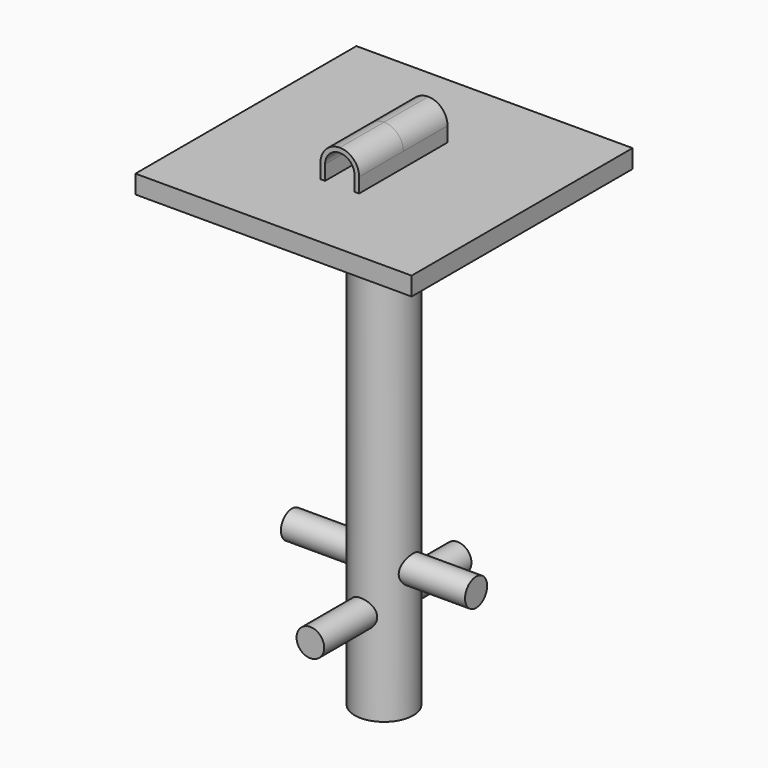
from build123d import *

# Parameters (mm, degrees)
F0_W     = 150
F0_H     = 150
F1_DEPTH = 10
F2_R     = 15.875
F2_R_2   = 13.375
F3_DEPTH = 250
F4_R     = 7.5
F5_DEPTH = 50
F6_R     = 7.5
F7_DEPTH = 50
F9_DEPTH = 30


# Not quite as in the source:
# - a feature names something its author has since deleted; it is built from what else it names


with BuildPart() as f1:
    # F0 (on Top) → F1 (new body)
    with BuildSketch(Plane.XY):
        Rectangle(F0_W, F0_H)
    extrude(amount=-F1_DEPTH)

    # F2 (on face) → F3 (join)
    with BuildSketch(Plane(origin=(0, 0, -10), x_dir=(1, 0, 0), z_dir=(0, 0, -1))):
        Circle(F2_R)
        Circle(F2_R_2, mode=Mode.SUBTRACT)
    extrude(amount=F3_DEPTH)

    # F4 (on Front) → F5 (join, symmetric)
    with BuildSketch(Plane.XZ):
        with Locations((0, -210)):
            Circle(F4_R)
    extrude(amount=F5_DEPTH, both=True)

    # F6 (on Right) → F7 (join, symmetric)
    with BuildSketch(Plane.YZ):
        with Locations((0, -190)):
            Circle(F6_R)
    extrude(amount=F7_DEPTH, both=True)

    # F8 (on Front) → F9 (join, symmetric)
    with BuildSketch(Plane.XZ):
        with BuildLine():
            Line((-10.5, 8), (-10.5, 0))
            Line((-10.5, 0), (-8, 0))
            Line((-8, 0), (-8, 8))
            ThreePointArc((-8, 8), (-5.6568542495, 13.6568542495), (0, 16))
            ThreePointArc((0, 16), (5.6568542495, 13.6568542495), (8, 8))
            Line((8, 8), (8, 0))
            Line((8, 0), (10.5, 0))
            Line((10.5, 0), (10.5, 8))
            ThreePointArc((10.5, 8), (7.4246212025, 15.4246212025), (0, 18.5))
            ThreePointArc((0, 18.5), (-7.4246212025, 15.4246212025), (-10.5, 8))
        make_face()
    extrude(amount=F9_DEPTH, both=True)


solid = f1.part
